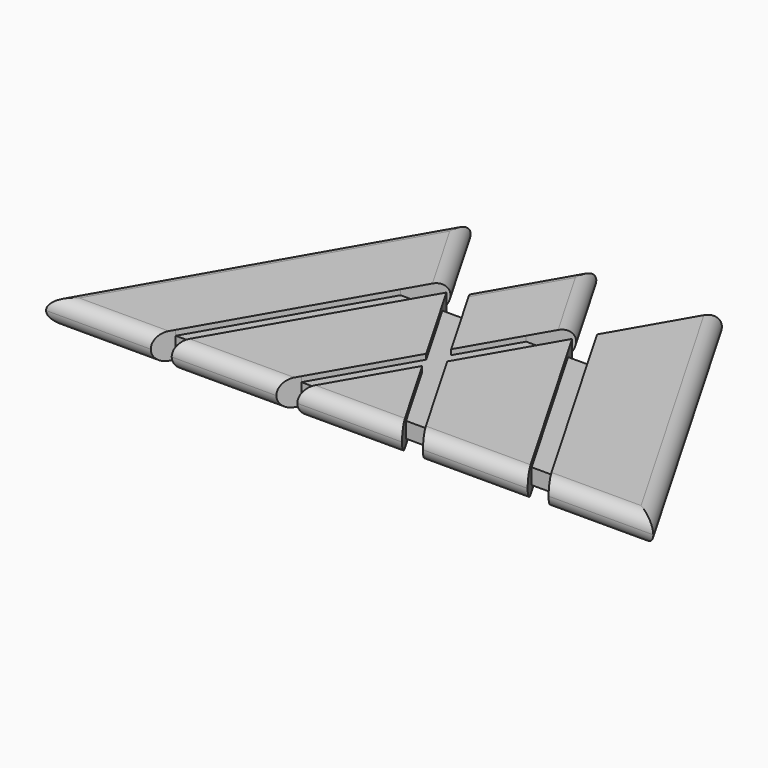
from build123d import *

# Parameters (mm, degrees)
F1_DEPTH = 3.175
F2_DEPTH = 1.905
F3_R     = 3.17499
F3_2_R   = 3.17499
F3_3_R   = 3.17499
F3_4_R   = 3.17499
F3_5_R   = 3.17499
F3_6_R   = 3.17499


# Not quite as in the source:
# - a fillet or chamfer is up to 0.001 mm smaller than in the source, because OpenCascade refuses the exact size


with BuildPart() as f1:
    # F0 (on Top) → F1 (new body, symmetric)
    with BuildSketch(Plane.XY):
        Polygon((43.18, 74.7899538708), (0, 0), (25.4, 0), (27.94, 4.3994090512), (50.8, 43.9940905122), (55.88, 52.7929086147), align=None)
    extrude(amount=F1_DEPTH, both=True)

    # F3 (radius 3.175 in the source; OpenCascade refuses exactly that, so slightly less here)
    f3_edges = [f1.edges().sort_by_distance(p)[0] for p in [
        (21.59, 37.394977, 3.175),
        (21.59, 37.394977, -3.175),
        (12.7, 0, -3.175),
        (12.7, 0, 3.175),
        (49.53, 63.791431, 3.175),
        (49.53, 63.791431, -3.175),
    ]]
    fillet(f3_edges, radius=F3_R)


with BuildPart() as f1b:
    # F0 (on Top) → F1, piece 2 (new body, symmetric)
    with BuildSketch(Plane.XY):
        Polygon((55.88, 43.9940905122), (33.02, 4.3994090512), (30.48, 0), (55.88, 0), (58.42, 4.3994090512), (71.12, 26.3964543073), (60.96, 43.9940905122), (58.42, 48.3934995635), align=None)
    extrude(amount=F1_DEPTH, both=True)

    # F3#3 (radius 3.175 in the source; OpenCascade refuses exactly that, so slightly less here)
    f3_3_edges = [f1b.edges().sort_by_distance(p)[0] for p in [
        (43.18, 0, -3.175),
        (43.18, 0, 3.175),
    ]]
    fillet(f3_3_edges, radius=F3_3_R)


with BuildPart() as f1c:
    # F0 (on Top) → F1, piece 3 (new body, symmetric)
    with BuildSketch(Plane.XY):
        Polygon((60.9602140859, 52.792537807), (66.04, 43.9940905122), (73.6602140859, 30.7954925508), (81.2823551529, 43.9952028573), (86.3618197643, 52.79161069), (73.6618197643, 74.7886559461), align=None)
    extrude(amount=F1_DEPTH, both=True)

    # F3#2 (radius 3.175 in the source; OpenCascade refuses exactly that, so slightly less here)
    f3_2_edges = [f1c.edges().sort_by_distance(p)[0] for p in [
        (67.311017, 63.790597, 3.175),
        (80.01182, 63.790133, 3.175),
        (80.01182, 63.790133, -3.175),
        (67.311017, 63.790597, -3.175),
    ]]
    fillet(f3_2_edges, radius=F3_2_R)


with BuildPart() as f1d:
    # F0 (on Top) → F1, piece 4 (new body, symmetric)
    with BuildSketch(Plane.XY):
        Polygon((88.9005352487, 48.3944264851), (86.360214113, 43.9952028573), (76.1989295703, 26.398308346), (88.9, 4.3994090512), (91.44, 0), (116.84, 0), (114.300072982, 4.3994511866), (91.4404622667, 43.9949752986), align=None)
    extrude(amount=F1_DEPTH, both=True)

    # F3#5 (radius 3.175 in the source; OpenCascade refuses exactly that, so slightly less here)
    f3_5_edges = [f1d.edges().sort_by_distance(p)[0] for p in [
        (104.14, 0, -3.175),
        (104.14, 0, 3.175),
    ]]
    fillet(f3_5_edges, radius=F3_5_R)


with BuildPart() as f1e:
    # F0 (on Top) → F1, piece 5 (new body, symmetric)
    with BuildSketch(Plane.XY):
        Polygon((73.66, 21.9970452561), (63.5, 4.3994090512), (60.96, 0), (86.36, 0), (83.82, 4.3994090512), align=None)
    extrude(amount=F1_DEPTH, both=True)

    # F3#4 (radius 3.175 in the source; OpenCascade refuses exactly that, so slightly less here)
    f3_4_edges = [f1e.edges().sort_by_distance(p)[0] for p in [
        (73.66, 0, -3.175),
        (73.66, 0, 3.175),
    ]]
    fillet(f3_4_edges, radius=F3_4_R)


with BuildPart() as f1f:
    # F0 (on Top) → F1, piece 6 (new body, symmetric)
    with BuildSketch(Plane.XY):
        Polygon((91.4408563844, 52.793650113), (96.520559582, 43.9949752986), (119.3800827134, 4.3994511866), (121.92, 0), (147.32, 0), (104.1424620628, 74.7897682521), align=None)
    extrude(amount=F1_DEPTH, both=True)

    # F3#6 (radius 3.175 in the source; OpenCascade refuses exactly that, so slightly less here)
    f3_6_edges = [f1f.edges().sort_by_distance(p)[0] for p in [
        (134.62, 0, -3.175),
        (125.731231, 37.394884, -3.175),
        (97.791659, 63.791709, -3.175),
        (134.62, 0, 3.175),
        (125.731231, 37.394884, 3.175),
    ]]
    fillet(f3_6_edges, radius=F3_6_R)


with BuildPart() as f2:
    # F0 (on Top) → F2 (new body, symmetric)
    with BuildSketch(Plane.XY):
        Polygon((96.520559582, 43.9949752986), (91.4404622667, 43.9949752986), (114.300072982, 4.3994511866), (119.3800827134, 4.3994511866), align=None)
    extrude(amount=F2_DEPTH, both=True)


with BuildPart() as f2b:
    # F0 (on Top) → F2, piece 2 (new body, symmetric)
    with BuildSketch(Plane.XY):
        Polygon((66.04, 43.9940905122), (60.96, 43.9940905122), (71.12, 26.3964543073), (58.42, 4.3994090512), (63.5, 4.3994090512), (73.66, 21.9970452561), (83.82, 4.3994090512), (88.9, 4.3994090512), (76.1989295703, 26.398308346), (86.360214113, 43.9952028573), (81.2823551529, 43.9952028573), (73.6602140859, 30.7954925508), align=None)
    extrude(amount=F2_DEPTH, both=True)


with BuildPart() as f2c:
    # F0 (on Top) → F2, piece 3 (new body, symmetric)
    with BuildSketch(Plane.XY):
        Polygon((50.8, 43.9940905122), (27.94, 4.3994090512), (33.02, 4.3994090512), (55.88, 43.9940905122), align=None)
    extrude(amount=F2_DEPTH, both=True)


solid = Compound([f1.part, f1b.part, f1c.part, f1d.part, f1e.part, f1f.part, f2.part, f2b.part, f2c.part])
